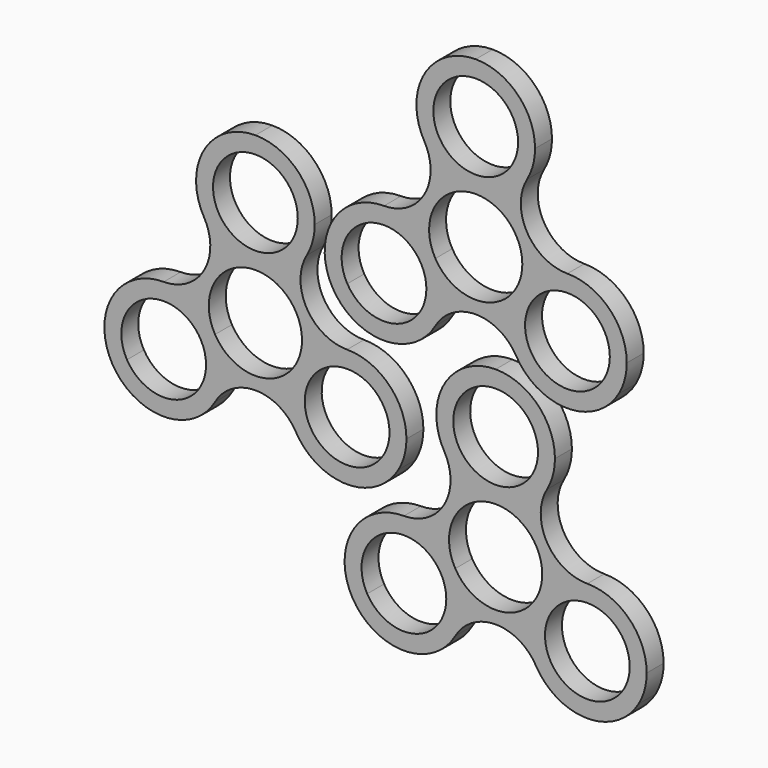
from build123d import *

# Parameters (mm, degrees)
F1_DEPTH = 5
F3_DEPTH = 5
F4_R     = 2.49999


# Not quite as in the source:
# - a fillet or chamfer is up to 0.001 mm smaller than in the source, because OpenCascade refuses the exact size
# - ends of sketch curves that miss each other by under 0.0002 mm in the source are joined


with BuildPart() as f1:
    # F0 (on Front) → F1 (new body)
    with BuildSketch(Plane.XZ):
        with BuildLine():
            ThreePointArc((38.5714030349, -38.744897142), (29.0454892287, -33.2484457762), (29.0506890964, -22.2505375922))
            ThreePointArc((29.0506890964, -22.2505375922), (23.9271254582, -27.3676448924), (16.9322220325, -29.2403481634))
            ThreePointArc((16.9322220325, -29.2403481634), (24.7103966204, -32.4621735732), (27.9322220245, -40.2403481634))
            ThreePointArc((27.9322220245, -40.2403481634), (27.5571071939, -43.0884730093), (26.4573465449, -45.7423480608))
            ThreePointArc((26.4573465449, -45.7423480608), (31.5776821767, -40.6220110514), (38.5714030349, -38.744897142))
        make_face()
        with BuildLine():
            ThreePointArc((26.4529371419, -59.7398014934), (38.5758217781, -66.7448936636), (50.7031171742, -59.7474402273))
            ThreePointArc((50.7031171742, -59.7474402273), (52.102812779, -56.3697808297), (52.5802317359, -52.7448943582))
            ThreePointArc((52.5802317359, -52.7448943582), (48.4766047631, -42.8422784964), (38.5714030349, -38.744897142))
            ThreePointArc((38.5714030349, -38.744897142), (31.5776821767, -40.6220110514), (26.4573465449, -45.7423480608))
            ThreePointArc((26.4573465449, -45.7423480608), (24.5802324305, -52.7404841531), (26.4529371419, -59.7398014934))
        make_face()
        with BuildLine():
            ThreePointArc((48.5802317359, -52.7448943582), (48.2392181953, -55.3340989807), (47.2394356204, -57.7467128361))
            ThreePointArc((47.2394356204, -57.7467128361), (28.9212452765, -50.1556897357), (48.5802317359, -52.7448943582))
        make_face(mode=Mode.SUBTRACT)
        with BuildLine():
            ThreePointArc((7.4115076436, -59.739801651), (16.9322223472, -54.2403481634), (26.4529371419, -59.7398014934))
            ThreePointArc((26.4529371419, -59.7398014934), (24.5802324305, -52.7404841531), (26.4573465449, -45.7423480608))
            ThreePointArc((26.4573465449, -45.7423480608), (16.9322223629, -51.2403481634), (7.4070978426, -45.7423486469))
            ThreePointArc((7.4070978426, -45.7423486469), (8.8067939707, -49.1200079519), (9.2842129657, -52.7448945972))
            ThreePointArc((9.2842129657, -52.7448945972), (8.8079351881, -56.3655212666), (7.4115076436, -59.739801651))
        make_face()
        with BuildLine():
            ThreePointArc((-4.7069607008, -38.7448971409), (-16.8386710918, -45.7423454469), (-16.8386731252, -59.7474402273))
            ThreePointArc((-16.8386731252, -59.7474402273), (-4.7113774064, -66.7448941415), (7.4115076436, -59.739801651))
            ThreePointArc((7.4115076436, -59.739801651), (8.8079351881, -56.3655212666), (9.2842129657, -52.7448945972))
            ThreePointArc((9.2842129657, -52.7448945972), (8.8067939707, -49.1200079519), (7.4070982561, -45.742348408))
            ThreePointArc((7.4070982561, -45.742348408), (2.2867615977, -40.622010617), (-4.7069607008, -38.7448971409))
        make_face()
        with BuildLine():
            ThreePointArc((5.284212727, -52.7448945972), (-2.1265828505, -62.4038811102), (-13.3749913647, -57.7467127167))
            ThreePointArc((-13.3749913647, -57.7467127167), (-7.3049916956, -43.0859080842), (5.284212727, -52.7448945972))
        make_face(mode=Mode.SUBTRACT)
        with BuildLine():
            ThreePointArc((16.9322220325, -29.2403481634), (9.9373177761, -27.3676444226), (4.8137540028, -22.2505359503))
            ThreePointArc((4.8137540028, -22.2505359503), (4.8189531712, -33.2484447192), (-4.7069607008, -38.7448971409))
            ThreePointArc((-4.7069607008, -38.7448971409), (2.2867615977, -40.622010617), (7.4070982561, -45.742348408))
            ThreePointArc((7.4070982561, -45.742348408), (7.4053651125, -34.7413484927), (16.9322220325, -29.2403481634))
        make_face()
        with BuildLine():
            ThreePointArc((30.9322220245, -15.2403481634), (26.8317169611, -5.3408532268), (16.9322220245, -1.2403481634))
            ThreePointArc((16.9322220245, -1.2403481634), (4.8049257674, -8.2454439116), (4.8137540028, -22.2505359503))
            ThreePointArc((4.8137540028, -22.2505359503), (9.9373177761, -27.3676444226), (16.9322220325, -29.2403481634))
            ThreePointArc((16.9322220325, -29.2403481634), (23.9271254582, -27.3676448924), (29.0506890964, -22.2505375922))
            ThreePointArc((29.0506890964, -22.2505375922), (30.4536594297, -18.8694982701), (30.9322220245, -15.2403481634))
        make_face()
        with BuildLine():
            ThreePointArc((26.9322220245, -15.2403481634), (9.8611542126, -22.3114159753), (16.9322220245, -5.2403481634))
            ThreePointArc((16.9322220245, -5.2403481634), (24.0032898364, -8.1692803516), (26.9322220245, -15.2403481634))
        make_face(mode=Mode.SUBTRACT)
    extrude(amount=F1_DEPTH)


with BuildPart() as f3:
    # F2 (on Front) → F3 (new body)
    with BuildSketch(Plane.XZ):
        with BuildLine():
            ThreePointArc((-45.6811212599, 50.1104917154), (-49.7816263233, 60.009986652), (-59.6811212599, 64.1104917154))
            Line((-59.6811212599, 64.1104917154), (-59.6811212599, 61.1104917154))
            ThreePointArc((-59.6811212599, 61.1104917154), (-51.9029466669, 57.8886663084), (-48.6811212599, 50.1104917154))
            ThreePointArc((-48.6811212599, 50.1104917154), (-51.9029466669, 42.3323171223), (-59.6811212599, 39.1104917154))
            ThreePointArc((-59.6811212599, 39.1104917154), (-56.4407509107, 38.7303301872), (-53.3763611535, 37.6104917154))
            ThreePointArc((-53.3763611535, 37.6104917154), (-50.5821641966, 39.4705208339), (-48.3110293727, 41.9421987189))
            ThreePointArc((-48.3110293727, 41.9421987189), (-46.3548073206, 45.8198790797), (-45.6811212599, 50.1104917154))
        make_face()
        with BuildLine():
            ThreePointArc((-65.9858813664, 37.6104917154), (-68.7800783233, 39.4705208339), (-71.0512131472, 41.9421987189))
            ThreePointArc((-71.0512131472, 41.9421987189), (-69.6565531618, 37.6104917154), (-71.0512131472, 33.2787847118))
            ThreePointArc((-71.0512131472, 33.2787847118), (-68.7800783233, 35.7504625969), (-65.9858813664, 37.6104917154))
        make_face()
        with BuildLine():
            Line((-59.6811212599, 61.1104917154), (-59.6811212599, 64.1104917154))
            ThreePointArc((-59.6811212599, 64.1104917154), (-72.1381695048, 56.49969738), (-71.0512131472, 41.9421987189))
            ThreePointArc((-71.0512131472, 41.9421987189), (-68.7800783233, 39.4705208339), (-65.9858813664, 37.6104917154))
            ThreePointArc((-65.9858813664, 37.6104917154), (-62.9214916091, 38.7303301872), (-59.6811212599, 39.1104917154))
            ThreePointArc((-59.6811212599, 39.1104917154), (-70.6811212599, 50.1104917154), (-59.6811212599, 61.1104917154))
        make_face()
        with BuildLine():
            Line((-59.6811212599, 36.1104917154), (-59.6811212599, 39.1104917154))
            ThreePointArc((-59.6811212599, 39.1104917154), (-62.9214916091, 38.7303301872), (-65.9858813664, 37.6104917154))
            ThreePointArc((-65.9858813664, 37.6104917154), (-62.9214916091, 36.4906532435), (-59.6811212599, 36.1104917154))
        make_face()
        with BuildLine():
            ThreePointArc((-53.3763611535, 37.6104917154), (-56.4407509107, 38.7303301872), (-59.6811212599, 39.1104917154))
            Line((-59.6811212599, 39.1104917154), (-59.6811212599, 36.1104917154))
            ThreePointArc((-59.6811212599, 36.1104917154), (-56.4407509107, 36.4906532435), (-53.3763611535, 37.6104917154))
        make_face()
        with BuildLine():
            ThreePointArc((-53.3763611535, 37.6104917154), (-56.4407509107, 36.4906532435), (-59.6811212599, 36.1104917154))
            ThreePointArc((-59.6811212599, 36.1104917154), (-51.9029466669, 32.8886663084), (-48.6811212599, 25.1104917154))
            ThreePointArc((-48.6811212599, 25.1104917154), (-51.9029466669, 17.3323171223), (-59.6811212599, 14.1104917154))
            ThreePointArc((-59.6811212599, 14.1104917154), (-56.4407509107, 13.7303301872), (-53.3763611535, 12.6104917154))
            ThreePointArc((-53.3763611535, 12.6104917154), (-50.5821641966, 14.4705208339), (-48.3110293727, 16.9421987189))
            ThreePointArc((-48.3110293727, 16.9421987189), (-46.3548073206, 20.8198790797), (-45.6811212599, 25.1104917154))
            ThreePointArc((-45.6811212599, 25.1104917154), (-46.3548073206, 29.401104351), (-48.3110293727, 33.2787847118))
            ThreePointArc((-48.3110293727, 33.2787847118), (-50.5821641966, 35.7504625969), (-53.3763611535, 37.6104917154))
        make_face()
        with BuildLine():
            ThreePointArc((-48.3110293727, 33.2787847118), (-49.705689358, 37.6104917154), (-48.3110293727, 41.9421987189))
            ThreePointArc((-48.3110293727, 41.9421987189), (-50.5821641966, 39.4705208339), (-53.3763611535, 37.6104917154))
            ThreePointArc((-53.3763611535, 37.6104917154), (-50.5821641966, 35.7504625969), (-48.3110293727, 33.2787847118))
        make_face()
        with BuildLine():
            ThreePointArc((-59.6811212599, 36.1104917154), (-62.9214916091, 36.4906532435), (-65.9858813664, 37.6104917154))
            ThreePointArc((-65.9858813664, 37.6104917154), (-68.7800783233, 35.7504625969), (-71.0512131472, 33.2787847118))
            ThreePointArc((-71.0512131472, 33.2787847118), (-73.6811212599, 25.1104917154), (-71.0512131472, 16.9421987189))
            ThreePointArc((-71.0512131472, 16.9421987189), (-68.7800783233, 14.4705208339), (-65.9858813664, 12.6104917154))
            ThreePointArc((-65.9858813664, 12.6104917154), (-62.9214916091, 13.7303301872), (-59.6811212599, 14.1104917154))
            ThreePointArc((-59.6811212599, 14.1104917154), (-67.459295853, 17.3323171223), (-70.6811212599, 25.1104917154))
            ThreePointArc((-70.6811212599, 25.1104917154), (-67.459295853, 32.8886663084), (-59.6811212599, 36.1104917154))
        make_face()
        with BuildLine():
            ThreePointArc((-59.6811212599, 14.1104917154), (-62.9214916091, 13.7303301872), (-65.9858813664, 12.6104917154))
            ThreePointArc((-65.9858813664, 12.6104917154), (-62.9214916091, 11.4906532435), (-59.6811212599, 11.1104917154))
            Line((-59.6811212599, 11.1104917154), (-59.6811212599, 14.1104917154))
        make_face()
        with BuildLine():
            ThreePointArc((-53.3763611535, 12.6104917154), (-56.4407509107, 13.7303301872), (-59.6811212599, 14.1104917154))
            Line((-59.6811212599, 14.1104917154), (-59.6811212599, 11.1104917154))
            ThreePointArc((-59.6811212599, 11.1104917154), (-56.4407509107, 11.4906532435), (-53.3763611535, 12.6104917154))
        make_face()
        with BuildLine():
            ThreePointArc((-48.3110293727, 8.2787847118), (-49.705689358, 12.6104917154), (-48.3110293727, 16.9421987189))
            ThreePointArc((-48.3110293727, 16.9421987189), (-50.5821641966, 14.4705208339), (-53.3763611535, 12.6104917154))
            ThreePointArc((-53.3763611535, 12.6104917154), (-50.5821641966, 10.7504625969), (-48.3110293727, 8.2787847118))
        make_face()
        with BuildLine():
            ThreePointArc((-53.3763611535, 12.6104917154), (-56.4407509107, 11.4906532435), (-59.6811212599, 11.1104917154))
            ThreePointArc((-59.6811212599, 11.1104917154), (-51.9029466669, 7.8886663084), (-48.6811212599, 0.1104917154))
            ThreePointArc((-48.6811212599, 0.1104917154), (-51.9029466669, -7.6676828777), (-59.6811212599, -10.8895082846))
            Line((-59.6811212599, -10.8895082846), (-59.6811212599, -13.8895082846))
            ThreePointArc((-59.6811212599, -13.8895082846), (-49.7816263233, -9.7890032212), (-45.6811212599, 0.1104917154))
            ThreePointArc((-45.6811212599, 0.1104917154), (-46.3548073206, 4.401104351), (-48.3110293727, 8.2787847118))
            ThreePointArc((-48.3110293727, 8.2787847118), (-50.5821641966, 10.7504625969), (-53.3763611535, 12.6104917154))
        make_face()
        with BuildLine():
            ThreePointArc((-65.9858813664, 12.6104917154), (-68.7800783233, 14.4705208339), (-71.0512131472, 16.9421987189))
            ThreePointArc((-71.0512131472, 16.9421987189), (-69.6565531618, 12.6104917154), (-71.0512131472, 8.2787847118))
            ThreePointArc((-71.0512131472, 8.2787847118), (-68.7800783233, 10.7504625969), (-65.9858813664, 12.6104917154))
        make_face()
        with BuildLine():
            ThreePointArc((-59.6811212599, 11.1104917154), (-62.9214916091, 11.4906532435), (-65.9858813664, 12.6104917154))
            ThreePointArc((-65.9858813664, 12.6104917154), (-68.7800783233, 10.7504625969), (-71.0512131472, 8.2787847118))
            ThreePointArc((-71.0512131472, 8.2787847118), (-72.1381695048, -6.2787139493), (-59.6811212599, -13.8895082846))
            Line((-59.6811212599, -13.8895082846), (-59.6811212599, -10.8895082846))
            ThreePointArc((-59.6811212599, -10.8895082846), (-70.6811212599, 0.1104917154), (-59.6811212599, 11.1104917154))
        make_face()
    extrude(amount=F3_DEPTH)

    # F4 (radius 2.5 in the source; OpenCascade refuses exactly that, so slightly less here)
    f4_edges = [f3.edges().sort_by_distance(p)[0] for p in [
        (-59.681121, -5, 64.110492),
        (-69.656553, -5, 37.610492),
        (-73.681121, -5, 25.110492),
        (-59.681121, 0, 64.110492),
        (-45.681121, 0, 25.110492),
        (-49.705689, 0, 12.610492),
        (-59.681121, 0, -13.889508),
        (-69.656553, 0, 12.610492),
        (-73.681121, 0, 25.110492),
        (-69.656553, 0, 37.610492),
        (-49.705689, 0, 37.610492),
        (-49.705689, -5, 37.610492),
        (-45.681121, -5, 25.110492),
        (-49.705689, -5, 12.610492),
        (-59.681121, -5, -13.889508),
        (-69.656553, -5, 12.610492),
    ]]
    fillet(f4_edges, radius=F4_R)


with BuildPart() as f5_1:
    # F5: copy of F1
    add(f1.part.moved(Location((-4.7, 0, 62.9))))


with BuildPart() as f6_1:
    # F6: copy of F5_1
    add(f5_1.part.moved(Location((-52, 0, -32.7))))


solid = Compound([f1.part, f5_1.part, f6_1.part])
